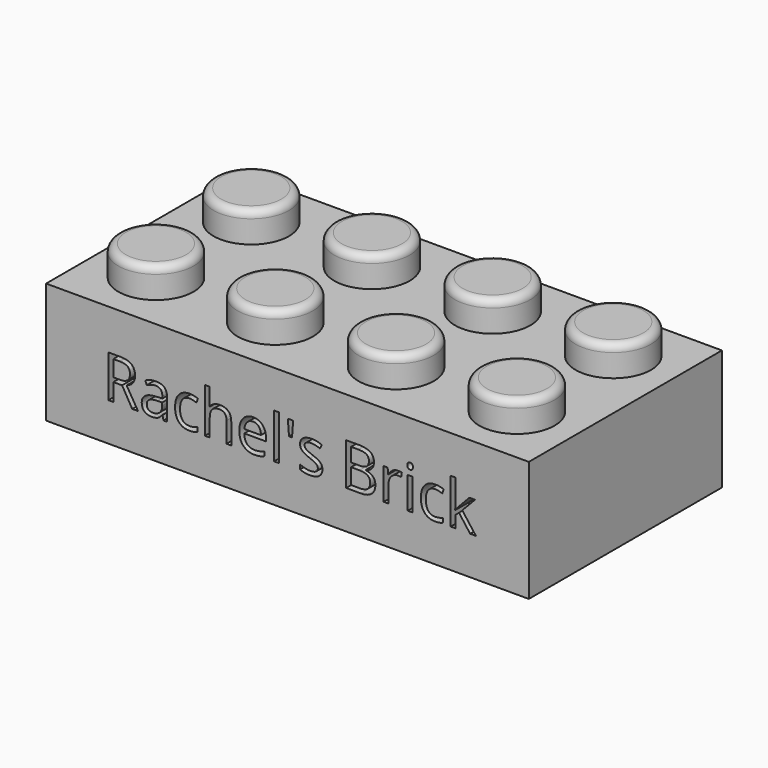
from build123d import *

# Parameters (mm, degrees)
F0_W         = 32
F0_H         = 16
F1_DEPTH     = 8
F3_T         = -1.5
F4_R         = 2.5
F5_DEPTH     = 2
F6_R         = 0.5
F7_R         = 3
F7_R_2       = 2.25
F8_DEPTH     = 7.8
F9_TEXT_SIZE = 3.9058685675
F10_DEPTH    = 2.25


# Not quite as in the source:
# - Text() gives the source's letters only with a copy of the font that has no kerning and outlines rounded to 1/6400 em; it was checked with that copy


with BuildPart() as f1:
    # F0 (on Top) → F1 (new body)
    with BuildSketch(Plane.XY):
        with Locations((-26.9199622543, -38.2962375879)):
            Rectangle(F0_W, F0_H)
    extrude(amount=F1_DEPTH)

    # F3
    f3_openings = [f1.faces().sort_by_distance(p)[0] for p in [
        (-26.919962, -38.296238, 0),
    ]]
    offset(amount=F3_T, openings=f3_openings)

    # F4 (on face) → F5 (join)
    with BuildSketch(Plane.XY.offset(8)):
        with Locations((-38.8813335449, -42.2388799489)):
            Circle(F4_R)
        with Locations((-30.9191979468, -42.3027127981)):
            Circle(F4_R)
        with Locations((-22.9191742837, -42.2956757247)):
            Circle(F4_R)
        with Locations((-14.9158546701, -42.2871597111)):
            Circle(F4_R)
        with Locations((-38.9199622543, -34.2962375879)):
            Circle(F4_R)
        with Locations((-30.9138204902, -34.3026593328)):
            Circle(F4_R)
        with Locations((-22.9155793786, -34.2969745398)):
            Circle(F4_R)
        with Locations((-14.9200959131, -34.2990793288)):
            Circle(F4_R)
    extrude(amount=F5_DEPTH)

    # F6
    f6_edges = [f1.edges().sort_by_distance(p)[0] for p in [
        (-41.381334, -42.23888, 10),
        (-41.419962, -34.296238, 10),
        (-33.419198, -42.302713, 10),
        (-33.41382, -34.302659, 10),
        (-25.419174, -42.295676, 10),
        (-25.415579, -34.296975, 10),
        (-17.415855, -42.28716, 10),
        (-17.420096, -34.299079, 10),
    ]]
    fillet(f6_edges, radius=F6_R)

    # F7 (on Top) → F8 (join)
    with BuildSketch(Plane.XY):
        with Locations((-34.9477143884, -38.2167436182)):
            Circle(F7_R)
        with Locations((-34.9477143884, -38.2167436182)):
            Circle(F7_R_2, mode=Mode.SUBTRACT)
        with Locations((-26.9477143884, -38.2167436182)):
            Circle(F7_R)
        with Locations((-26.9477143884, -38.2167436182)):
            Circle(F7_R_2, mode=Mode.SUBTRACT)
        with Locations((-18.9477143884, -38.2167436182)):
            Circle(F7_R)
        with Locations((-18.9477143884, -38.2167436182)):
            Circle(F7_R_2, mode=Mode.SUBTRACT)
    extrude(amount=F8_DEPTH)

    # F9 (on face) → F10 (cut)
    with BuildSketch(Plane.XZ.offset(46.2962375879)):
        with Locations((-39.1727839974, 2.5388741099)):
            Text("Rachel's Brick", F9_TEXT_SIZE, font='Open Sans', text_align=(TextAlign.LEFT, TextAlign.BOTTOM))
    extrude(amount=-F10_DEPTH, mode=Mode.SUBTRACT)


solid = f1.part
